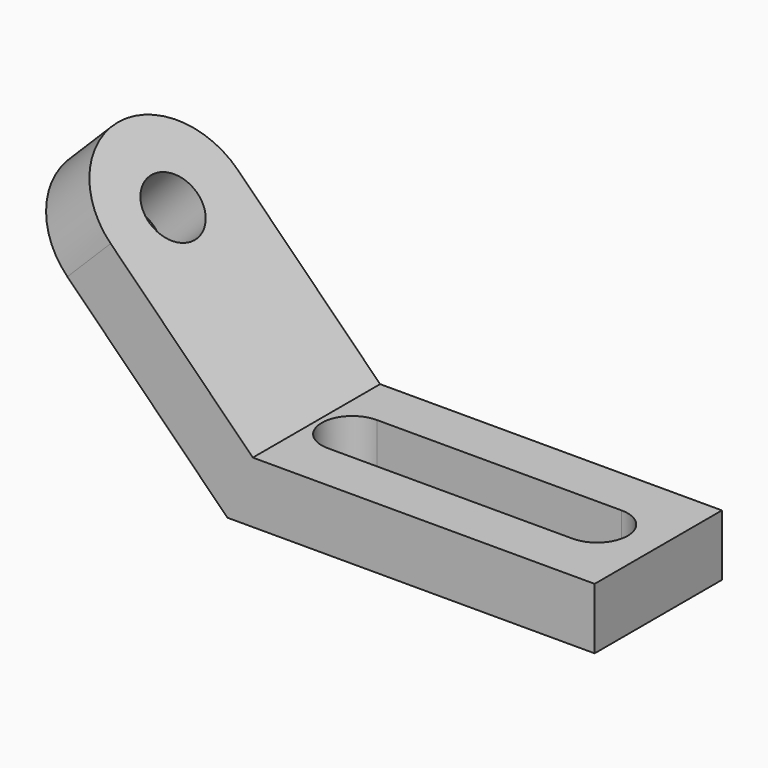
from build123d import *

# Parameters (mm, degrees)
F1_DEPTH = 52
F3_DEPTH = 20
F5_DEPTH = 25
F6_R     = 26
F7_R     = 25.99999


# Not quite as in the source:
# - a fillet or chamfer is up to 0.001 mm smaller than in the source, because OpenCascade refuses the exact size


with BuildPart() as f1:
    # F0 (on Front) → F1 (new body)
    with BuildSketch(Plane.XZ):
        Polygon((-38.2547932683, -20), (-38.2547932683, 0), (-35.5326342583, 0), (-29.9705220208, 0), (-94.8233357632, 64.8528137424), (-108.9654713869, 50.7106781187), align=None)
        Polygon((-35.5326342583, 0), (-38.2547932683, 0), (-38.2547932683, -20), (-9.9705220208, -20), (-29.9705220208, 0), align=None)
        Polygon((81.7452067317, 0), (-29.9705220208, 0), (-9.9705220208, -20), (81.7452067317, -20), align=None)
    extrude(amount=F1_DEPTH)

    # F2 (on face) → F3 (cut)
    with BuildSketch(Plane.XY):
        with BuildLine():
            Line((-18.2547932683, -36), (61.7452067317, -36))
            ThreePointArc((61.7452067317, -36), (68.8162745436, -33.0710678119), (71.7452067317, -26))
            ThreePointArc((71.7452067317, -26), (68.8162745436, -18.9289321881), (61.7452067317, -16))
            Line((61.7452067317, -16), (-18.2547932683, -16))
            ThreePointArc((-18.2547932683, -16), (-28.2547932683, -26), (-18.2547932683, -36))
        make_face()
    extrude(amount=-F3_DEPTH, mode=Mode.SUBTRACT)

    # F4 (on face) → F5 (cut)
    with BuildSketch(Plane(origin=(-14.9852610104, 0, -14.9852610104), x_dir=(0, 1, 0), z_dir=(0.7071067812, 0, 0.7071067812))):
        with BuildLine():
            ThreePointArc((-16.4961378883, 86.9204033326), (-19.2517821929, 93.8138285014), (-26, 96.9080881091))
            Line((-26, 96.9080881091), (-26.9922757766, 96.9080881091))
            ThreePointArc((-26.9922757766, 96.9080881091), (-33.3895630572, 79.6760476372), (-16.4961378883, 86.9204033326))
        make_face()
    extrude(amount=-F5_DEPTH, mode=Mode.SUBTRACT)

    # F6
    f6_edges = [f1.edges().sort_by_distance(p)[0] for p in [
        (-101.894404, -52, 57.781746),
    ]]
    fillet(f6_edges, radius=F6_R)

    # F7 (radius 26 in the source; OpenCascade refuses exactly that, so slightly less here)
    f7_edges = [f1.edges().sort_by_distance(p)[0] for p in [
        (-101.894404, 0, 57.781746),
    ]]
    fillet(f7_edges, radius=F7_R)


solid = f1.part
